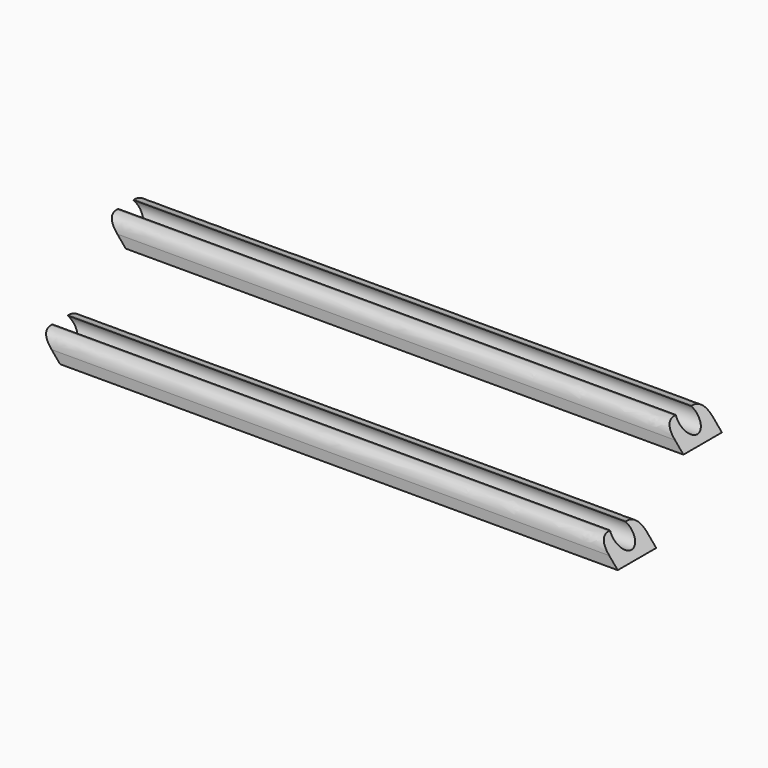
from build123d import *

# Parameters (mm, degrees)
F0_W        = 180
F0_H        = 15
F1_DEPTH    = 7.15
F3_DEPTH    = 180
F4_T1_DEPTH = 51.8569072778
F5_T1_DEPTH = 41.3548246674
F5_T3_DEPTH = 41.3548246674
F6_T1_DEPTH = 194.0004376371


# Not quite as in the source:
# - a fillet or chamfer that OpenCascade refuses, or shapes differently, is made with other operations: its cross-section is extruded or revolved along the edge and cut away or added


with BuildPart() as f1:
    # F0 (on Top) → F1 (new body)
    with BuildSketch(Plane.XY):
        Rectangle(F0_W, F0_H)
    extrude(amount=F1_DEPTH)

    # F2 (on face) → F3 (cut)
    with BuildSketch(Plane(origin=(-90, 0, 0), x_dir=(0, -1, 0), z_dir=(-1, 0, 0))):
        with BuildLine():
            ThreePointArc((-3.0020826105, 7.15), (-0.8790093839, 2.1138581411), (3.45, 5.45))
            ThreePointArc((3.45, 5.45), (3.3361418589, 6.3290093839), (3.0020826105, 7.15))
            Line((3.0020826105, 7.15), (-3.0020826105, 7.15))
        make_face()
    extrude(amount=-F3_DEPTH, mode=Mode.SUBTRACT)

    # F4: chamfer of 7.15 x 5.9995623629 on 1 edges, made by hand

    # F4_s2 → F4_t1 (cut)
    with BuildSketch(Plane.XZ.offset(-25.9284536389)):
        Polygon((-84.0004376371, 0), (-90, 7.15), (-90, 0), align=None)
    extrude(amount=F4_T1_DEPTH, mode=Mode.SUBTRACT)

    # F5: chamfer of 7.15 x 5.9995623629 on 2 edges, made by hand

    # F5_s2 → F5_t1 (cut)
    with BuildSketch(Plane.XZ.offset(-15.4263710285)):
        Polygon((90, 0), (84.0004376371, 7.15), (90, 7.15), align=None)
    extrude(amount=F5_T1_DEPTH, mode=Mode.SUBTRACT)

    # F5_s4 → F5_t3 (cut)
    with BuildSketch(Plane.XZ.offset(-25.9284536389)):
        Polygon((90, 0), (84.0004376371, 7.15), (90, 7.15), align=None)
    extrude(amount=F5_T3_DEPTH, mode=Mode.SUBTRACT)

    # F6: fillet of radius 4 on 2 edges, made by hand

    # F6_s2 → F6_t1 (cut)
    with BuildSketch(Plane.YZ.offset(-100)):
        with BuildLine():
            add(Edge.make_bspline(
                [(-7.5, 3.15), (-7.5, 7.15), (-3.5, 7.15)],
                knots=[0, 0, 0, 1, 1, 1], degree=2, weights=[1, 1, 1]))
            Line((-3.5, 7.15), (-7.5, 7.15))
            Line((-7.5, 7.15), (-7.5, 3.15))
        make_face()
        with BuildLine():
            add(Edge.make_bspline(
                [(7.5, 3.15), (7.5, 7.15), (3.5, 7.15)],
                knots=[0, 0, 0, 1, 1, 1], degree=2, weights=[1, 1, 1]))
            Line((3.5, 7.15), (7.5, 7.15))
            Line((7.5, 7.15), (7.5, 3.15))
        make_face()
    extrude(amount=F6_T1_DEPTH, mode=Mode.SUBTRACT)


with BuildPart() as f7_1:
    # F7: copy of F1
    add(f1.part.moved(Location((0, 37.9, 0))))


with BuildPart() as f9_1:
    # F9: copy of F1
    add(f1.part.moved(Location((20.5, 0, 38.4))))


solid = Compound([f1.part, f9_1.part])
